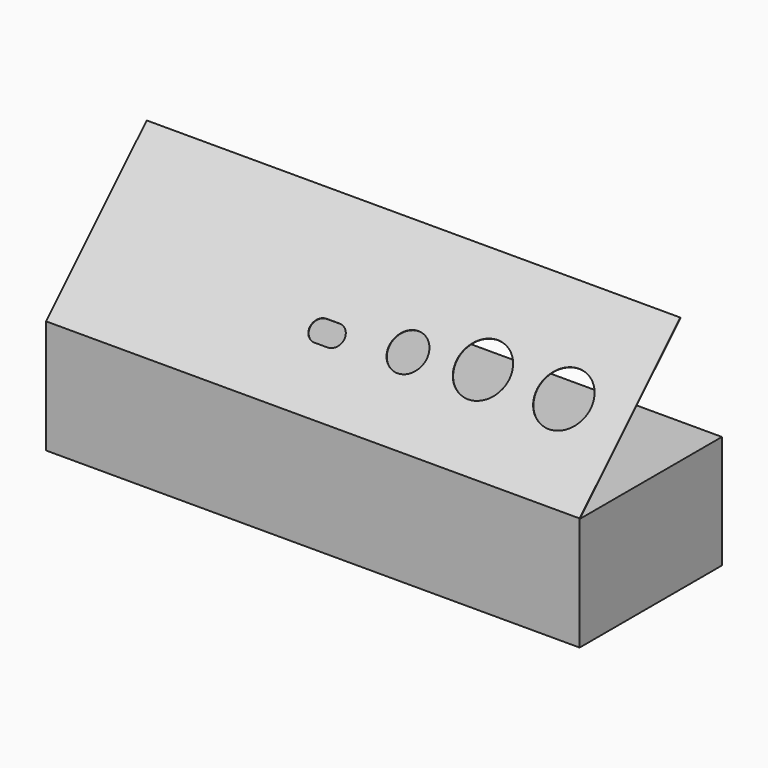
from build123d import *

# Parameters (mm, degrees)
F1_DEPTH = 209.55
F3_DEPTH = 0.4064


# Not quite as in the source:
# - the dataset's text gives a spline's control points without its knots; the knots are read off the source's solid


with BuildPart() as f1:
    # F0 (on Right) → F1 (new body, symmetric)
    with BuildSketch(Plane.YZ):
        Polygon((-139.7, 0), (0, 0), (0, 88.9), (-139.2936, 88.9), (-139.2936, 89.154), (-40.6298144724, 187.8177855276), (-40.9171826682, 188.1051537235), (-139.7, 89.3223363917), align=None)
    extrude(amount=F1_DEPTH, both=True)

    # F2 (on face) → F3 (cut, through all)
    with BuildSketch(Plane(origin=(0, -114.5111681959, 114.5111681959), x_dir=(1, 0, 0), z_dir=(0, -0.7071067812, 0.7071067812))):
        with BuildLine():
            add(Edge.make_bspline(
                [(-30.4346554714, 12.4755289708), (-28.8919356714, 10.9324789708), (-26.7232582714, 10.0343349708), (-24.5415760714, 10.0343349708)],
                knots=[3, 3, 3, 3, 4, 4, 4, 4], degree=3))
            Line((-24.5415760714, 10.0343349708), (-14.2228260714, 10.0343349708))
            add(Edge.make_bspline(
                [(-14.2228260714, 10.0343349708), (-12.0402548714, 10.0343349708), (-9.8723140714, 10.9324789708), (-8.3296196714, 12.4755289708)],
                knots=[0, 0, 0, 0, 1, 1, 1, 1], degree=3))
            add(Edge.make_bspline(
                [(-8.3296196714, 12.4755289708), (-6.7864680714, 14.0182741708), (-5.8884256714, 16.1866213708), (-5.8884256714, 18.3687099708), (-5.8884256714, 20.5508747708), (-6.7864680714, 22.7191711708), (-8.3296196714, 24.2622719708)],
                knots=[1, 1, 1, 1, 2, 2, 2, 3, 3, 3, 3], degree=3))
            add(Edge.make_bspline(
                [(-8.3296196714, 24.2622719708), (-9.8723140714, 25.8049663708), (-12.0402548714, 26.7030849708), (-14.2228260714, 26.7030849708)],
                knots=[3, 3, 3, 3, 4, 4, 4, 4], degree=3))
            Line((-14.2228260714, 26.7030849708), (-24.5415760714, 26.7030849708))
            add(Edge.make_bspline(
                [(-24.5415760714, 26.7030849708), (-26.7232582714, 26.7030849708), (-28.8919356714, 25.8049663708), (-30.4346554714, 24.2622719708)],
                knots=[0, 0, 0, 0, 1, 1, 1, 1], degree=3))
            add(Edge.make_bspline(
                [(-30.4346554714, 24.2622719708), (-31.9773752714, 22.7191711708), (-32.8759510714, 20.5508747708), (-32.8759510714, 18.3687099708), (-32.8759510714, 16.1866213708), (-31.9773752714, 14.0182741708), (-30.4346554714, 12.4755289708)],
                knots=[1, 1, 1, 1, 2, 2, 2, 3, 3, 3, 3], degree=3))
        make_face()
        with BuildLine():
            add(Edge.make_bspline(
                [(50.9739701286, 35.1022299708), (48.2554589286, 37.8204363708), (44.4345115286, 39.4030849708), (40.5900437286, 39.4030849708)],
                knots=[7, 7, 7, 7, 8, 8, 8, 8], degree=3))
            add(Edge.make_bspline(
                [(40.5900437286, 39.4030849708), (36.7460839286, 39.4030849708), (32.9251365286, 37.8204363708), (30.2066253286, 35.1022299708)],
                knots=[0, 0, 0, 0, 1, 1, 1, 1], degree=3))
            add(Edge.make_bspline(
                [(30.2066253286, 35.1022299708), (27.4884189286, 32.3837441708), (25.9056687286, 28.5627713708), (25.9056687286, 24.7187099708), (25.9056687286, 20.8743691708), (27.4884189286, 17.0535741708), (30.2066253286, 14.3355455708)],
                knots=[1, 1, 1, 1, 2, 2, 2, 3, 3, 3, 3], degree=3))
            add(Edge.make_bspline(
                [(30.2066253286, 14.3355455708), (32.9251365286, 11.6170089708), (36.7460839286, 10.0343349708), (40.5900437286, 10.0343349708), (44.4345115286, 10.0343349708), (48.2554589286, 11.6170089708), (50.9739701286, 14.3355455708)],
                knots=[3, 3, 3, 3, 4, 4, 4, 5, 5, 5, 5], degree=3))
            add(Edge.make_bspline(
                [(50.9739701286, 14.3355455708), (53.6921765286, 17.0535741708), (55.2744187286, 20.8743691708), (55.2744187286, 24.7187099708), (55.2744187286, 28.5627713708), (53.6921765286, 32.3837441708), (50.9739701286, 35.1022299708)],
                knots=[5, 5, 5, 5, 6, 6, 6, 7, 7, 7, 7], degree=3))
        make_face()
        with BuildLine():
            add(Edge.make_bspline(
                [(110.7016129286, 45.2649223708), (106.8809957286, 49.0851839708), (101.5114865286, 51.3095127708), (96.1084493286, 51.3095127708)],
                knots=[7, 7, 7, 7, 8, 8, 8, 8], degree=3))
            add(Edge.make_bspline(
                [(96.1084493286, 51.3095127708), (90.7062757286, 51.3095127708), (85.3364109286, 49.0851839708), (81.5161493286, 45.2649223708)],
                knots=[0, 0, 0, 0, 1, 1, 1, 1], degree=3))
            add(Edge.make_bspline(
                [(81.5161493286, 45.2649223708), (77.6955067286, 41.4443305708), (75.4709493286, 36.0747705708), (75.4709493286, 30.6720127708), (75.4709493286, 25.2692549708), (77.6955067286, 19.8992123708), (81.5161493286, 16.0789507708)],
                knots=[1, 1, 1, 1, 2, 2, 2, 3, 3, 3, 3], degree=3))
            add(Edge.make_bspline(
                [(81.5161493286, 16.0789507708), (85.3364109286, 12.2585113708), (90.7062757286, 10.0345127708), (96.1084493286, 10.0345127708), (101.5114865286, 10.0345127708), (106.8809957286, 12.2585113708), (110.7016129286, 16.0789507708)],
                knots=[3, 3, 3, 3, 4, 4, 4, 5, 5, 5, 5], degree=3))
            add(Edge.make_bspline(
                [(110.7016129286, 16.0789507708), (114.5218745286, 19.8992123708), (116.7459493286, 25.2692549708), (116.7459493286, 30.6720127708), (116.7459493286, 36.0747705708), (114.5218745286, 41.4443305708), (110.7016129286, 45.2649223708)],
                knots=[5, 5, 5, 5, 6, 6, 6, 7, 7, 7, 7], degree=3))
        make_face()
        with BuildLine():
            add(Edge.make_bspline(
                [(174.3060069286, 45.9422641708), (170.4119075286, 49.8362111708), (164.9391219286, 52.1032627708), (159.4321479286, 52.1032627708)],
                knots=[7, 7, 7, 7, 8, 8, 8, 8], degree=3))
            add(Edge.make_bspline(
                [(159.4321479286, 52.1032627708), (153.9258597286, 52.1032627708), (148.4526169286, 49.8362111708), (144.5589747286, 45.9422641708)],
                knots=[0, 0, 0, 0, 1, 1, 1, 1], degree=3))
            add(Edge.make_bspline(
                [(144.5589747286, 45.9422641708), (140.6649769286, 42.0482663708), (138.3976713286, 36.5757347708), (138.3976713286, 31.0688877708), (138.3976713286, 25.5620661708), (140.6649769286, 20.0890519708), (144.5589747286, 16.1950541708), (148.4526169286, 12.3014119708), (153.9258597286, 10.0345127708), (159.4321479286, 10.0345127708), (164.9391219286, 10.0345127708), (170.4119075286, 12.3014119708), (174.3060069286, 16.1950541708)],
                knots=[1, 1, 1, 1, 2, 2, 2, 3, 3, 3, 4, 4, 4, 5, 5, 5, 5], degree=3))
            add(Edge.make_bspline(
                [(174.3060069286, 16.1950541708), (178.1996491286, 20.0890519708), (180.4665229286, 25.5620661708), (180.4665229286, 31.0688877708), (180.4665229286, 36.5757347708), (178.1996491286, 42.0482663708), (174.3060069286, 45.9422641708)],
                knots=[5, 5, 5, 5, 6, 6, 6, 7, 7, 7, 7], degree=3))
        make_face()
    extrude(amount=-F3_DEPTH, mode=Mode.SUBTRACT)


solid = f1.part
